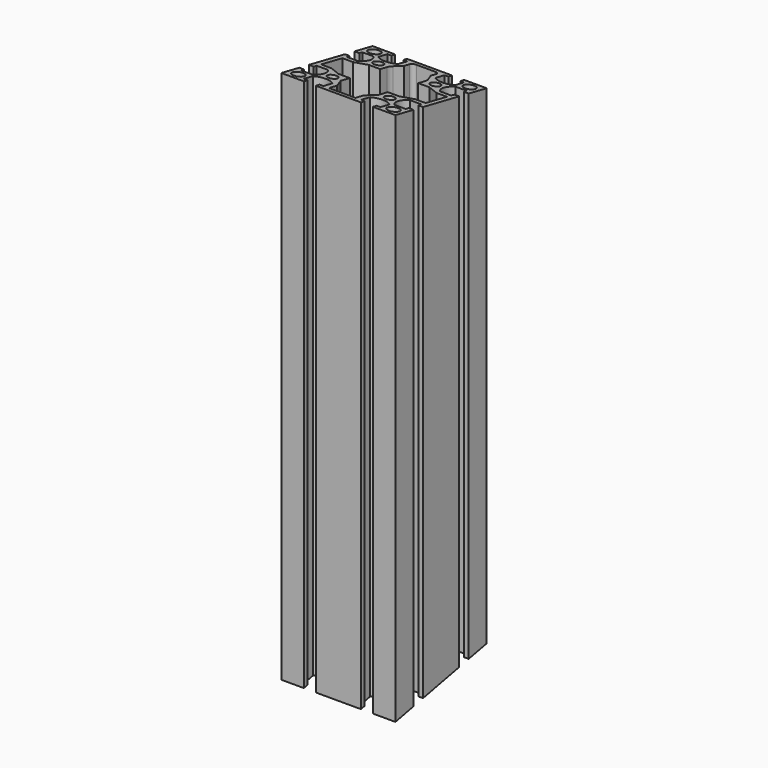
from build123d import *

# Parameters (mm, degrees)
F0_R          = 3
F0_R_2        = 2.5
F1_DEPTH      = 280.86
F2_R          = 2
F3_R          = 7
F6_DEPTH      = 30
F6_DEPTH_BACK = 30


# Not quite as in the source:
# - a feature names something its author has since deleted; it is built from what else it names


with BuildPart() as f1:
    # F0 (on Top) → F1 (new body)
    with BuildSketch(Plane.XY):
        with BuildLine():
            Line((18.15, -30), (30, -30))
            Line((30, -30), (30, -18.15))
            Line((30, -18.15), (27.5, -18.15))
            Line((27.5, -18.15), (27.5, -20.15))
            Line((27.5, -20.15), (21.5477069044, -20.15))
            ThreePointArc((21.5477069044, -20.15), (19.5, -15), (21.5477069044, -9.85))
            Line((21.5477069044, -9.85), (27.5, -9.85))
            Line((27.5, -9.85), (27.5, -11.85))
            Line((27.5, -11.85), (30, -11.85))
            Line((30, -11.85), (30, 11.85))
            Line((30, 11.85), (27.5, 11.85))
            Line((27.5, 11.85), (27.5, 9.85))
            Line((27.5, 9.85), (21.5477069044, 9.85))
            ThreePointArc((21.5477069044, 9.85), (19.5, 15), (21.5477069044, 20.15))
            Line((21.5477069044, 20.15), (27.5, 20.15))
            Line((27.5, 20.15), (27.5, 18.15))
            Line((27.5, 18.15), (30, 18.15))
            Line((30, 18.15), (30, 30))
            Line((30, 30), (18.15, 30))
            Line((18.15, 30), (18.15, 27.5))
            Line((18.15, 27.5), (20.15, 27.5))
            Line((20.15, 27.5), (20.15, 21.5477069044))
            ThreePointArc((20.15, 21.5477069044), (15, 19.5), (9.85, 21.5477069044))
            Line((9.85, 21.5477069044), (9.85, 27.5))
            Line((9.85, 27.5), (11.85, 27.5))
            Line((11.85, 27.5), (11.85, 30))
            Line((11.85, 30), (-11.85, 30))
            Line((-11.85, 30), (-11.85, 27.5))
            Line((-11.85, 27.5), (-9.85, 27.5))
            Line((-9.85, 27.5), (-9.85, 21.5477069044))
            ThreePointArc((-9.85, 21.5477069044), (-15, 19.5), (-20.15, 21.5477069044))
            Line((-20.15, 21.5477069044), (-20.15, 27.5))
            Line((-20.15, 27.5), (-18.15, 27.5))
            Line((-18.15, 27.5), (-18.15, 30))
            Line((-18.15, 30), (-30, 30))
            Line((-30, 30), (-30, 18.15))
            Line((-30, 18.15), (-27.5, 18.15))
            Line((-27.5, 18.15), (-27.5, 20.15))
            Line((-27.5, 20.15), (-21.5477069044, 20.15))
            ThreePointArc((-21.5477069044, 20.15), (-19.5, 15), (-21.5477069044, 9.85))
            Line((-21.5477069044, 9.85), (-27.5, 9.85))
            Line((-27.5, 9.85), (-27.5, 11.85))
            Line((-27.5, 11.85), (-30, 11.85))
            Line((-30, 11.85), (-30, -11.85))
            Line((-30, -11.85), (-27.5, -11.85))
            Line((-27.5, -11.85), (-27.5, -9.85))
            Line((-27.5, -9.85), (-21.5477069044, -9.85))
            ThreePointArc((-21.5477069044, -9.85), (-19.5, -15), (-21.5477069044, -20.15))
            Line((-21.5477069044, -20.15), (-27.5, -20.15))
            Line((-27.5, -20.15), (-27.5, -18.15))
            Line((-27.5, -18.15), (-30, -18.15))
            Line((-30, -18.15), (-30, -30))
            Line((-30, -30), (-18.15, -30))
            Line((-18.15, -30), (-18.15, -27.5))
            Line((-18.15, -27.5), (-20.15, -27.5))
            Line((-20.15, -27.5), (-20.15, -21.5477069044))
            ThreePointArc((-20.15, -21.5477069044), (-15, -19.5), (-9.85, -21.5477069044))
            Line((-9.85, -21.5477069044), (-9.85, -27.5))
            Line((-9.85, -27.5), (-11.85, -27.5))
            Line((-11.85, -27.5), (-11.85, -30))
            Line((-11.85, -30), (11.85, -30))
            Line((11.85, -30), (11.85, -27.5))
            Line((11.85, -27.5), (9.85, -27.5))
            Line((9.85, -27.5), (9.85, -21.5477069044))
            ThreePointArc((9.85, -21.5477069044), (15, -19.5), (20.15, -21.5477069044))
            Line((20.15, -21.5477069044), (20.15, -27.5))
            Line((20.15, -27.5), (18.15, -27.5))
            Line((18.15, -27.5), (18.15, -30))
        make_face()
        with Locations((-25, -25)):
            Circle(F0_R, mode=Mode.SUBTRACT)
        with Locations((-15, -15)):
            Circle(F0_R_2, mode=Mode.SUBTRACT)
        with Locations((25, -25)):
            Circle(F0_R, mode=Mode.SUBTRACT)
        with Locations((15, -15)):
            Circle(F0_R_2, mode=Mode.SUBTRACT)
        with Locations((-25, 25)):
            Circle(F0_R, mode=Mode.SUBTRACT)
        with Locations((-15, 15)):
            Circle(F0_R_2, mode=Mode.SUBTRACT)
        Polygon((-7, 22), (-7, 27.5), (0, 27.5), (7, 27.5), (7, 22), (10, 16), (10, 10), (16, 10), (22, 7), (27.5, 7), (27.5, 0), (27.5, -7), (22, -7), (16, -10), (10, -10), (10, -16), (7, -22), (7, -27.5), (0, -27.5), (-7, -27.5), (-7, -22), (-10, -16), (-10, -10), (-16, -10), (-22, -7), (-27.5, -7), (-27.5, 0), (-27.5, 7), (-22, 7), (-16, 10), (-10, 10), (-10, 16), align=None, mode=Mode.SUBTRACT)
        with Locations((15, 15)):
            Circle(F0_R_2, mode=Mode.SUBTRACT)
        with Locations((25, 25)):
            Circle(F0_R, mode=Mode.SUBTRACT)
    extrude(amount=F1_DEPTH)

    # F2
    f2_edges = [f1.edges().sort_by_distance(p)[0] for p in [
        (-7, 27.5, 140.43),
        (7, 27.5, 140.43),
    ]]
    fillet(f2_edges, radius=F2_R)

    # F3
    f3_edges = [f1.edges().sort_by_distance(p)[0] for p in [
        (-10, 16, 140.43),
        (10, 16, 140.43),
    ]]
    fillet(f3_edges, radius=F3_R)

    # F5 (on Right) → F6 (cut, two sides)
    with BuildSketch(Plane.YZ) as f6_sk:
        Polygon((166.5976946582, -66.7170951811), (146.3493769552, 35.0780720561), (-30, 0), (-9.751682297, -101.7951672372), align=None)
        Polygon((135.5963626007, 247.9208354856), (151.7094622056, 328.9268574701), (-13.8869003951, 361.8660219845), (-30, 280.86), align=None)
    extrude(amount=F6_DEPTH, mode=Mode.SUBTRACT)
    extrude(f6_sk.sketch, amount=-F6_DEPTH_BACK, mode=Mode.SUBTRACT)


solid = f1.part
